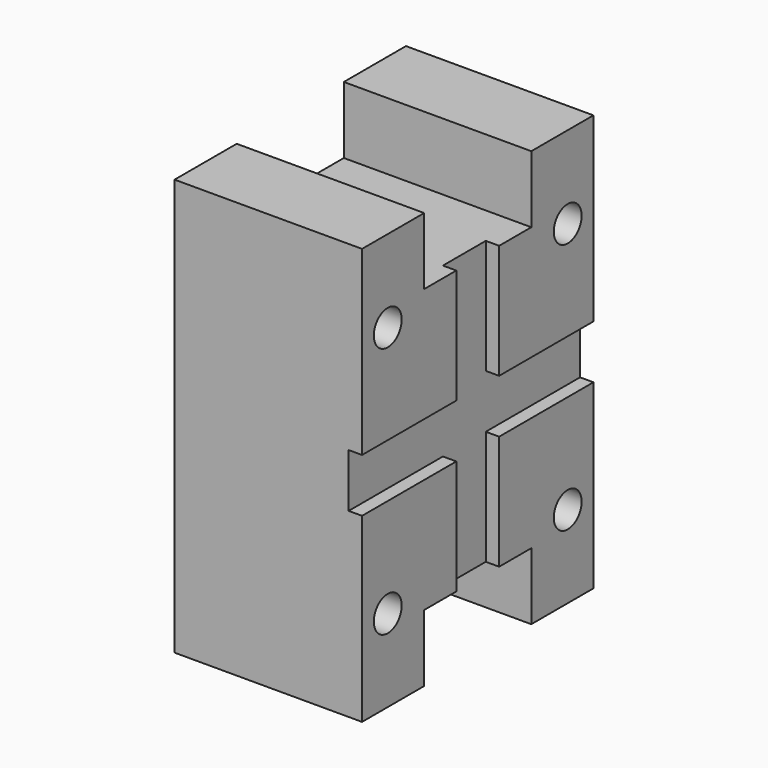
from build123d import *

# Parameters (mm, degrees)
F0_W     = 108
F0_H     = 155.5
F1_DEPTH = 70
F2_R     = 6.5
F3_DEPTH = 70.001
F4_W     = 50
F4_H     = 25
F5_DEPTH = 70.001
F6_R     = 10
F7_DEPTH = 20
F8_W     = 20
F8_H     = 42.75
F8_H_2   = 20
F8_W_2   = 44
F9_DEPTH = 5


with BuildPart() as f1:
    # F0 (on Right) → F1 (new body)
    with BuildSketch(Plane.YZ):
        Rectangle(F0_W, F0_H)
    extrude(amount=-F1_DEPTH)

    # F2 (on face) → F3 (cut, through all)
    with BuildSketch(Plane(origin=(-70, 0, 0), x_dir=(0, -1, 0), z_dir=(-1, 0, 0))):
        with Locations((-42, 47)):
            Circle(F2_R)
        with Locations((42, 47)):
            Circle(F2_R)
        with Locations((-42, -47)):
            Circle(F2_R)
        with Locations((42, -47)):
            Circle(F2_R)
    extrude(amount=-F3_DEPTH, mode=Mode.SUBTRACT)

    # F4 (on face) → F5 (cut, through all)
    with BuildSketch(Plane(origin=(-70, 0, 0), x_dir=(0, -1, 0), z_dir=(-1, 0, 0))):
        with Locations((0, 65.25)):
            Rectangle(F4_W, F4_H)
        with Locations((0, -65.25)):
            Rectangle(F4_W, F4_H)
    extrude(amount=-F5_DEPTH, mode=Mode.SUBTRACT)

    # F6 (on face) → F7 (cut)
    with BuildSketch(Plane(origin=(-70, 0, 0), x_dir=(0, -1, 0), z_dir=(-1, 0, 0))):
        with Locations((-42, 47)):
            Circle(F6_R)
        with Locations((-42, -47)):
            Circle(F6_R)
        with Locations((42, 47)):
            Circle(F6_R)
        with Locations((42, -47)):
            Circle(F6_R)
    extrude(amount=-F7_DEPTH, mode=Mode.SUBTRACT)

    # F8 (on face) → F9 (cut)
    with BuildSketch(Plane.YZ):
        with Locations((0, 31.375)):
            Rectangle(F8_W, F8_H)
        Rectangle(F8_W, F8_H_2)
        with Locations((-32, 0)):
            Rectangle(F8_W_2, F8_H_2)
        with Locations((32, 0)):
            Rectangle(F8_W_2, F8_H_2)
        with Locations((0, -31.375)):
            Rectangle(F8_W, F8_H)
    extrude(amount=-F9_DEPTH, mode=Mode.SUBTRACT)


solid = f1.part
